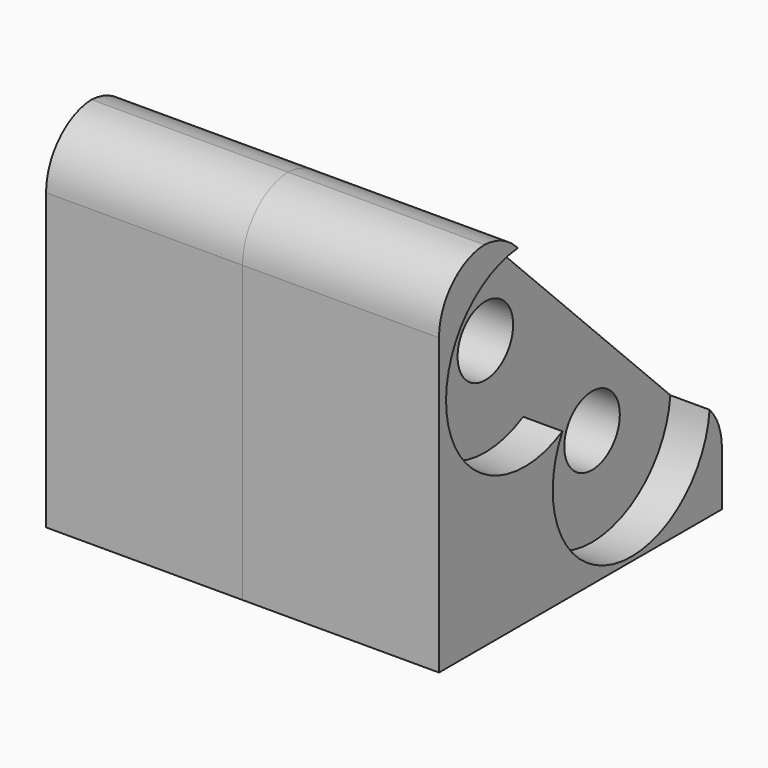
from build123d import *

# Parameters (mm, degrees)
F0_W        = 90
F0_H        = 90
F0_R        = 8.83
F1_DEPTH    = 50
F2_T1_DEPTH = 410.0356183152
F3_T1_DEPTH = 81.066017178
F3_T3_DEPTH = 125
F4_DEPTH    = 10
F6_DEPTH    = 10
F7_R        = 8.83
F8_DEPTH    = 10


# Not quite as in the source:
# - a fillet or chamfer that OpenCascade refuses, or shapes differently, is made with other operations: its cross-section is extruded or revolved along the edge and cut away or added


with BuildPart() as f1:
    # F0 (on Right) → F1 (new body)
    with BuildSketch(Plane.YZ):
        Rectangle(F0_W, F0_H)
        with BuildLine():
            ThreePointArc((-5.7369661858, -6.8994105845), (-39.269643101, 27.758238797), (7.242218534, 15.0208996323))
            ThreePointArc((7.242218534, 15.0208996323), (6.4600606697, 8.8163752919), (4.1625287508, 3.0000843521))
            ThreePointArc((4.1625287508, 3.0000843521), (28.9206831957, 2.5916357703), (41.1833440309, -18.9202258647))
            ThreePointArc((41.1833440309, -18.9202258647), (9.9788196906, -43.1380680004), (-5.7369661858, -6.8994105845))
        make_face(mode=Mode.SUBTRACT)
        with BuildLine():
            ThreePointArc((4.1625287508, 3.0000843521), (-0.0801119364, -2.6567698974), (-5.7369661858, -6.8994105845))
            ThreePointArc((-5.7369661858, -6.8994105845), (9.9788196906, -43.1380680004), (41.1833440309, -18.9202258647))
            ThreePointArc((41.1833440309, -18.9202258647), (28.9206831957, 2.5916357703), (4.1625287508, 3.0000843521))
        make_face()
        with Locations((16.1833440309, -18.9202258647)):
            Circle(F0_R, mode=Mode.SUBTRACT)
        with BuildLine():
            ThreePointArc((4.1625287508, 3.0000843521), (6.4600606697, 8.8163752919), (7.242218534, 15.0208996323))
            ThreePointArc((7.242218534, 15.0208996323), (-39.269643101, 27.758238797), (-5.7369661858, -6.8994105845))
            ThreePointArc((-5.7369661858, -6.8994105845), (-1.4943254987, -1.242556335), (4.1625287508, 3.0000843521))
        make_face()
        with Locations((-17.757781466, 15.0208996323)):
            Circle(F0_R, mode=Mode.SUBTRACT)
        with BuildLine():
            ThreePointArc((4.1625287508, 3.0000843521), (-1.4943254987, -1.242556335), (-5.7369661858, -6.8994105845))
            ThreePointArc((-5.7369661858, -6.8994105845), (-0.0801119364, -2.6567698974), (4.1625287508, 3.0000843521))
        make_face()
    extrude(amount=F1_DEPTH)

    # F2: chamfer of 70 on 1 edges, made by hand

    # F2_s2 → F2_t1 (cut)
    with BuildSketch(Plane.YZ.offset(-180.0178091576)):
        Polygon((45, -25), (-25, 45), (45, 45), align=None)
    extrude(amount=F2_T1_DEPTH, mode=Mode.SUBTRACT)

    # F3: fillet of radius 15 on 3 edges, made by hand

    # F3_s2 → F3_t1 (cut)
    with BuildSketch(Plane.YZ.offset(-15.533008589)):
        with BuildLine():
            ThreePointArc((45, -31.2132034356), (43.8581929877, -25.4729519501), (40.6066017178, -20.6066017178))
            Line((40.6066017178, -20.6066017178), (45, -25))
            Line((45, -25), (45, -31.2132034356))
        make_face()
        with BuildLine():
            ThreePointArc((-20.6066017178, 40.6066017178), (-25.4729519501, 43.8581929877), (-31.2132034356, 45))
            Line((-31.2132034356, 45), (-25, 45))
            Line((-25, 45), (-20.6066017178, 40.6066017178))
        make_face()
    extrude(amount=F3_T1_DEPTH, mode=Mode.SUBTRACT)

    # F3_s4 → F3_t3 (cut)
    with BuildSketch(Plane.YZ.offset(-37.5)):
        with BuildLine():
            ThreePointArc((-45, 30), (-40.6066017178, 40.6066017178), (-30, 45))
            Line((-30, 45), (-45, 45))
            Line((-45, 45), (-45, 30))
        make_face()
    extrude(amount=F3_T3_DEPTH, mode=Mode.SUBTRACT)

    # F0 (on Right) → F4 (cut)
    with BuildSketch(Plane.YZ):
        with BuildLine():
            ThreePointArc((4.1625287508, 3.0000843521), (6.4600606697, 8.8163752919), (7.242218534, 15.0208996323))
            ThreePointArc((7.242218534, 15.0208996323), (-39.269643101, 27.758238797), (-5.7369661858, -6.8994105845))
            ThreePointArc((-5.7369661858, -6.8994105845), (-1.4943254987, -1.242556335), (4.1625287508, 3.0000843521))
        make_face()
        with Locations((-17.757781466, 15.0208996323)):
            Circle(F0_R, mode=Mode.SUBTRACT)
        with BuildLine():
            ThreePointArc((4.1625287508, 3.0000843521), (-0.0801119364, -2.6567698974), (-5.7369661858, -6.8994105845))
            ThreePointArc((-5.7369661858, -6.8994105845), (9.9788196906, -43.1380680004), (41.1833440309, -18.9202258647))
            ThreePointArc((41.1833440309, -18.9202258647), (28.9206831957, 2.5916357703), (4.1625287508, 3.0000843521))
        make_face()
        with Locations((16.1833440309, -18.9202258647)):
            Circle(F0_R, mode=Mode.SUBTRACT)
        with BuildLine():
            ThreePointArc((4.1625287508, 3.0000843521), (-1.4943254987, -1.242556335), (-5.7369661858, -6.8994105845))
            ThreePointArc((-5.7369661858, -6.8994105845), (-0.0801119364, -2.6567698974), (4.1625287508, 3.0000843521))
        make_face()
    extrude(amount=F4_DEPTH, mode=Mode.SUBTRACT)

    # F5 (on face) → F6 (cut, through all)
    with BuildSketch(Plane.YZ):
        with BuildLine():
            ThreePointArc((4.1625287508, 3.0000843521), (8.9331762586, 5.0053894309), (14.014482738, 5.985517262))
            Line((14.014482738, 5.985517262), (7.1479616607, 12.8520383393))
            ThreePointArc((7.1479616607, 12.8520383393), (6.1678338296, 7.7707318599), (4.1625287508, 3.0000843521))
        make_face()
    extrude(amount=F6_DEPTH, mode=Mode.SUBTRACT)

    # F7 (on face) → F8 (join)
    with BuildSketch(Plane.YZ.offset(50)):
        with Locations((-17.757781466, 15.0208996323)):
            Circle(F7_R)
        with Locations((16.1833440309, -18.9202258647)):
            Circle(F7_R)
    extrude(amount=-F8_DEPTH)

    # F12: sweep along a path in F9
    with BuildLine(Plane(origin=(40, 0, 0), x_dir=(0, -1, 0), z_dir=(-1, 0, 0))) as f12_path:
        Line((17.757781466, 15.0208996323), (-52.1658341758, -50.6265266045))
    # F11 (on face) → F12 (sweep, cut)
    with BuildSketch(Plane(origin=(0, -10.4996791259, 9.8575696436), x_dir=(1, 0, 0), z_dir=(0, -0.7290478078, 0.6844627776))):
        with BuildLine():
            ThreePointArc((40, 3.796413521), (35, -1.203586479), (40, -6.203586479))
            Line((40, -6.203586479), (40, 3.796413521))
        make_face()
        with BuildLine():
            Line((40, 3.796413521), (40, -6.203586479))
            ThreePointArc((40, -6.203586479), (43.5355339059, -4.739120385), (45, -1.203586479))
            ThreePointArc((45, -1.203586479), (43.5355339059, 2.3319474269), (40, 3.796413521))
        make_face()
    sweep(path=f12_path.line, mode=Mode.SUBTRACT)


with BuildPart() as f13_1:
    # F13: instance of F1
    add(f1.part.mirror(Plane(origin=(50, -9.1492689096, -9.8684610313), x_dir=(0, 1, 0), z_dir=(1, 0, 0))))


solid = Compound([f1.part, f13_1.part])
